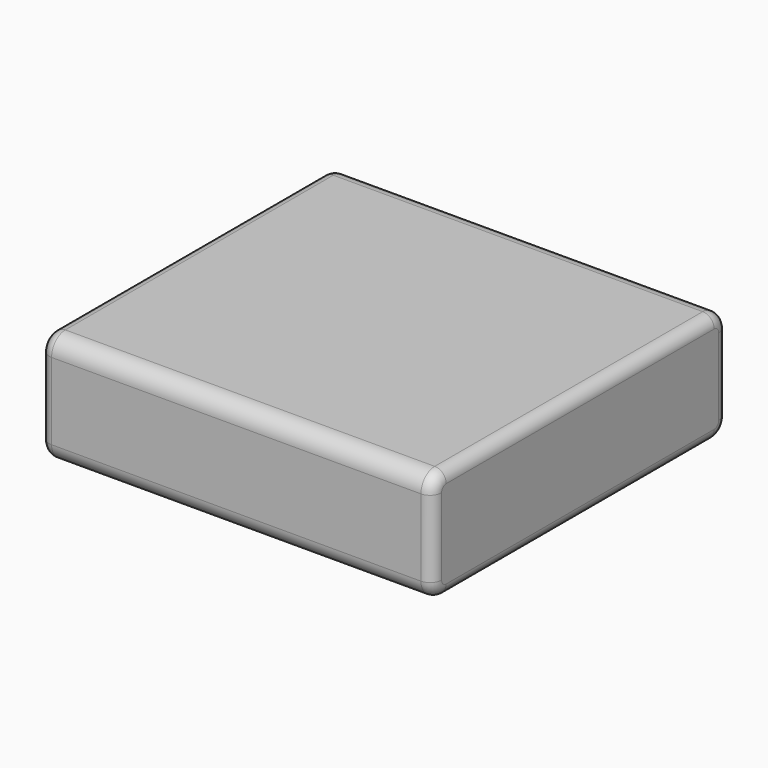
from build123d import *

# Parameters (mm, degrees)
F0_W          = 64.4
F0_H          = 68.4
F1_DEPTH      = 19.4
F2_R          = 3
F3_R          = 2
F4_W          = 8.2
F4_H          = 4.35
F5_DEPTH      = 2.5
F6_W          = 3
F6_H          = 3
F7_DEPTH      = 3.8
F8_R          = 1.78
F9_DEPTH      = 2
F10_TEXT_SIZE = 3.2406108841
F11_DEPTH     = 0.5
F14_ANGLE     = 180
F16_ANGLE     = 90


# Not quite as in the source:
# - Text() gives the source's letters only with a copy of the font that has no kerning and outlines rounded to 1/6400 em; it was checked with that copy


with BuildPart() as f1:
    # F0 (on Top) → F1 (new body)
    with BuildSketch(Plane.XY):
        Rectangle(F0_W, F0_H)
    extrude(amount=F1_DEPTH)

    # F2
    f2_edges = [f1.edges().sort_by_distance(p)[0] for p in [
        (-32.2, 0, 19.4),
        (32.2, 0, 19.4),
        (32.2, 0, 0),
        (-32.2, 0, 0),
    ]]
    fillet(f2_edges, radius=F2_R)

    # F3
    f3_edges = [f1.edges().sort_by_distance(p)[0] for p in [
        (-32.2, -34.2, 9.7),
        (-31.32132, -34.2, 0.87868),
        (-31.32132, -34.2, 18.52132),
        (0, -34.2, 0),
        (0, -34.2, 19.4),
        (31.32132, -34.2, 0.87868),
        (31.32132, -34.2, 18.52132),
        (32.2, -34.2, 9.7),
        (32.2, 34.2, 9.7),
        (31.32132, 34.2, 0.87868),
        (31.32132, 34.2, 18.52132),
        (0, 34.2, 0),
        (0, 34.2, 19.4),
        (-31.32132, 34.2, 0.87868),
        (-31.32132, 34.2, 18.52132),
        (-32.2, 34.2, 9.7),
    ]]
    fillet(f3_edges, radius=F3_R)

    # F4 (on face) → F5 (cut)
    with BuildSketch(Plane.XY.offset(19.4)):
        with Locations((20.6, 28.425)):
            Rectangle(F4_W, F4_H)
    extrude(amount=-F5_DEPTH, mode=Mode.SUBTRACT)

    # F6 (on face) → F7 (join)
    with BuildSketch(Plane.XY.offset(16.9)):
        with Locations((18.675, 28.425)):
            Rectangle(F6_W, F6_H)
    extrude(amount=F7_DEPTH)

    # F8 (on face) → F9 (cut)
    with BuildSketch(Plane(origin=(0, 34.2, 0), x_dir=(-1, 0, 0), z_dir=(0, 1, 0))):
        with Locations((24.26, 13.89)):
            Circle(F8_R)
    extrude(amount=-F9_DEPTH, mode=Mode.SUBTRACT)

    # F10 (on face) → F11 (join)
    with BuildSketch(Plane.XY.offset(19.4)):
        with Locations((14.715, 22.4167601635)):
            Text('OFF-ON', F10_TEXT_SIZE, font='Open Sans', text_align=(TextAlign.LEFT, TextAlign.BOTTOM))
    extrude(amount=F11_DEPTH)


with BuildPart() as f1_1:
    # F14: moved
    add(f1.part.rotate(Axis((0, 0.7596462965, 0), (0, -1, 0)), F14_ANGLE))


with BuildPart() as f1_2:
    # F16: moved
    add(f1_1.part.rotate(Axis((0, 0, 19.4975901395), (0, 0, 1)), F16_ANGLE))


solid = f1_2.part
